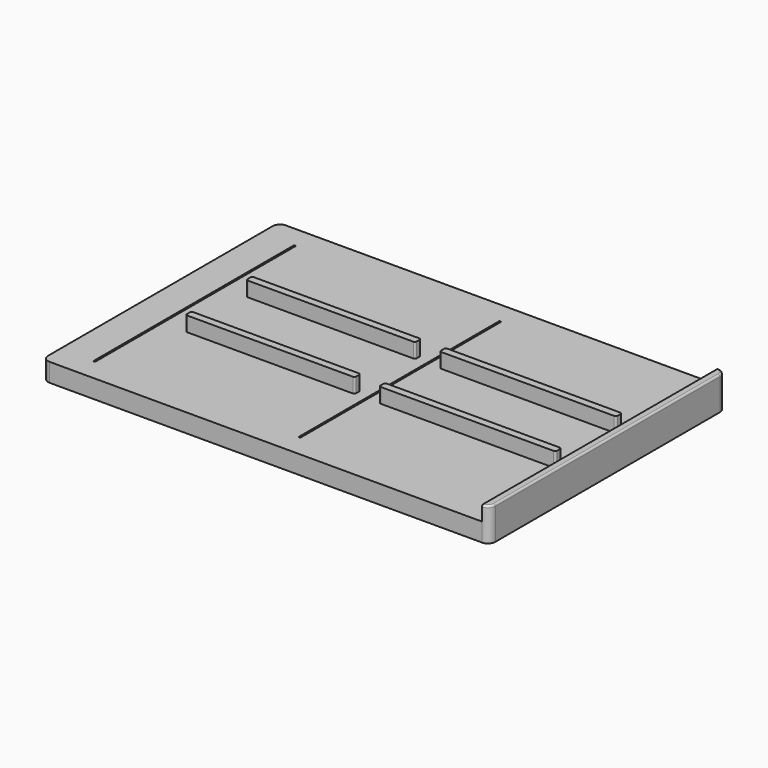
from build123d import *

# Parameters (mm, degrees)
F0_W         = 119.1
F0_H         = 80
F1_DEPTH     = 5
F3_DEPTH     = 63.1
F4_W         = 6.8
F4_H         = 2
F4_W_2       = 7
F4_W_3       = 6.5
F5_DEPTH     = 4
F6_W         = 47.8
F6_H         = 2
F7_DEPTH     = 4
F8_W         = 0.5
F8_H         = 68
F9_DEPTH     = 25
F10_W        = 80
F10_H        = 5
F11_DEPTH    = 2
F12_W        = 2
F12_H        = 32.5577612221
F12_H_2      = 47.4422387779
F13_DEPTH    = 4
F14_R        = 1.99999
F15_R        = 0.5
F16_R        = 0.1
F17_T1_DEPTH = 76.00002
F17_T3_DEPTH = 1.25001
F17_T6_ANGLE = 90
F17_T8_ANGLE = 90


# Not quite as in the source:
# - a fillet or chamfer that OpenCascade refuses, or shapes differently, is made with other operations: its cross-section is extruded or revolved along the edge and cut away or added
# - a fillet or chamfer is up to 0.001 mm smaller than in the source, because OpenCascade refuses the exact size


with BuildPart() as f1:
    # F0 (on Top) → F1 (new body)
    with BuildSketch(Plane.XY):
        with Locations((59.55, 40)):
            Rectangle(F0_W, F0_H)
    extrude(amount=F1_DEPTH)

    # F2 (on face) → F3 (cut)
    with BuildSketch(Plane.XY.offset(5)):
        Polygon((64.6, 74), (64.6, 25), (64.6, 6), (65.1, 6), (65.1, 74), align=None)
    extrude(amount=-F3_DEPTH, mode=Mode.SUBTRACT)

    # F4 (on face) → F5 (join)
    with BuildSketch(Plane.XY.offset(5)):
        with Locations((32.5, 50.25)):
            Rectangle(F4_W, F4_H)
        Polygon((35.9, 49.25), (39.1217214942, 49.25), (41.1, 49.25), (41.1, 51.25), (35.9, 51.25), align=None)
        with Locations((44.6, 50.25)):
            Rectangle(F4_W_2, F4_H)
        with Locations((51.35, 50.25)):
            Rectangle(F4_W_3, F4_H)
        with Locations((19.2, 50.25)):
            Rectangle(F4_W, F4_H)
        with Locations((25.85, 50.25)):
            Rectangle(F4_W_3, F4_H)
        with Locations((58.1, 50.25)):
            Rectangle(F4_W_2, F4_H)
        with Locations((44.6, 29.75)):
            Rectangle(F4_W_2, F4_H)
        with Locations((32.5, 29.75)):
            Rectangle(F4_W, F4_H)
        with Locations((58.1, 29.75)):
            Rectangle(F4_W_2, F4_H)
        Polygon((41.1, 30.75), (39.1217214942, 30.75), (35.9, 30.75), (35.9, 28.75), (39.8, 28.75), (41.1, 28.75), align=None)
        with Locations((51.35, 29.75)):
            Rectangle(F4_W_3, F4_H)
        with Locations((25.85, 29.75)):
            Rectangle(F4_W_3, F4_H)
        with Locations((19.2, 29.75)):
            Rectangle(F4_W, F4_H)
    extrude(amount=F5_DEPTH)

    # F6 (on face) → F7 (join)
    with BuildSketch(Plane.XY.offset(5)):
        with Locations((92.1, 50.25)):
            Rectangle(F6_W, F6_H)
        with Locations((92.1, 29.75)):
            Rectangle(F6_W, F6_H)
    extrude(amount=F7_DEPTH)

    # F8 (on face) → F9 (cut)
    with BuildSketch(Plane.XY.offset(5)):
        with Locations((9.25, 40)):
            Rectangle(F8_W, F8_H)
    extrude(amount=-F9_DEPTH, mode=Mode.SUBTRACT)

    # F10 (on face) → F11 (join)
    with BuildSketch(Plane.YZ.offset(119.1)):
        with Locations((40, 2.5)):
            Rectangle(F10_W, F10_H)
    extrude(amount=F11_DEPTH)

    # F12 (on face) → F13 (join)
    with BuildSketch(Plane.XY.offset(5)):
        with Locations((120.1, 63.7211193889)):
            Rectangle(F12_W, F12_H)
        with Locations((120.1, 23.7211193889)):
            Rectangle(F12_W, F12_H_2)
    extrude(amount=F13_DEPTH)

    # F14 (radius 2 in the source; OpenCascade refuses exactly that, so slightly less here)
    f14_edges = [f1.edges().sort_by_distance(p)[0] for p in [
        (0, 80, 2.5),
        (0, 0, 2.5),
        (121.1, 80, 4.5),
        (121.1, 0, 4.5),
    ]]
    fillet(f14_edges, radius=F14_R)

    # F15
    f15_edges = [f1.edges().sort_by_distance(p)[0] for p in [
        (15.8, 49.25, 7),
        (15.8, 51.25, 7),
        (61.6, 49.25, 7),
        (61.6, 51.25, 7),
        (68.2, 49.25, 7),
        (68.2, 51.25, 7),
        (116, 49.25, 7),
        (116, 51.25, 7),
        (116, 28.75, 7),
        (116, 30.75, 7),
        (68.2, 28.75, 7),
        (68.2, 30.75, 7),
        (61.6, 28.75, 7),
        (61.6, 30.75, 7),
        (15.8, 28.75, 7),
        (15.8, 30.75, 7),
    ]]
    fillet(f15_edges, radius=F15_R)

    # F16
    f16_edges = [f1.edges().sort_by_distance(p)[0] for p in [
        (9.5, 6, 2.5),
        (9, 6, 2.5),
        (9.5, 74, 2.5),
        (9, 74, 2.5),
        (64.6, 74, 2.5),
        (65.1, 74, 2.5),
        (64.6, 6, 2.5),
        (65.1, 6, 2.5),
    ]]
    fillet(f16_edges, radius=F16_R)

    # F17: fillet of radius 0.5 on 1 edges, made by hand

    # F17_s2 → F17_t1 (cut)
    with BuildSketch(Plane.XZ.offset(-78.00001)):
        with BuildLine():
            ThreePointArc((120.6, 9), (120.9535533906, 8.8535533906), (121.1, 8.5))
            Line((121.1, 8.5), (121.1, 9))
            Line((121.1, 9), (120.6, 9))
        make_face()
    extrude(amount=F17_T1_DEPTH, mode=Mode.SUBTRACT)

    # F17_s4 → F17_t3 (cut)
    with BuildSketch(Plane.YZ.offset(117.85)):
        with BuildLine():
            ThreePointArc((80, 8.5), (79.8535533906, 8.8535533906), (79.5, 9))
            Line((79.5, 9), (80, 9))
            Line((80, 9), (80, 8.5))
        make_face()
        with BuildLine():
            ThreePointArc((0, 8.5), (0.1464466094, 8.8535533906), (0.5, 9))
            Line((0.5, 9), (0, 9))
            Line((0, 9), (0, 8.5))
        make_face()
    extrude(amount=F17_T3_DEPTH, mode=Mode.SUBTRACT)

    # F17_s5 → F17_t6 (revolve, cut)
    with BuildSketch(Plane.XZ.offset(-1.99999)):
        with BuildLine():
            ThreePointArc((120.6, 9), (120.9535533906, 8.8535533906), (121.1, 8.5))
            Line((121.1, 8.5), (121.1, 9))
            Line((121.1, 9), (120.6, 9))
        make_face()
    revolve(axis=Axis((119.10001, 1.99999, 9), (0, 0, -1)), revolution_arc=F17_T6_ANGLE, mode=Mode.SUBTRACT)

    # F17_s7 → F17_t8 (revolve, cut)
    with BuildSketch(Plane.XZ.offset(-78.00001)):
        with BuildLine():
            ThreePointArc((121.1, 8.5), (120.9535533906, 8.8535533906), (120.6, 9))
            Line((120.6, 9), (121.1, 9))
            Line((121.1, 9), (121.1, 8.5))
        make_face()
    revolve(axis=Axis((119.10001, 78.00001, 9), (0, 0, 1)), revolution_arc=F17_T8_ANGLE, mode=Mode.SUBTRACT)


solid = f1.part
